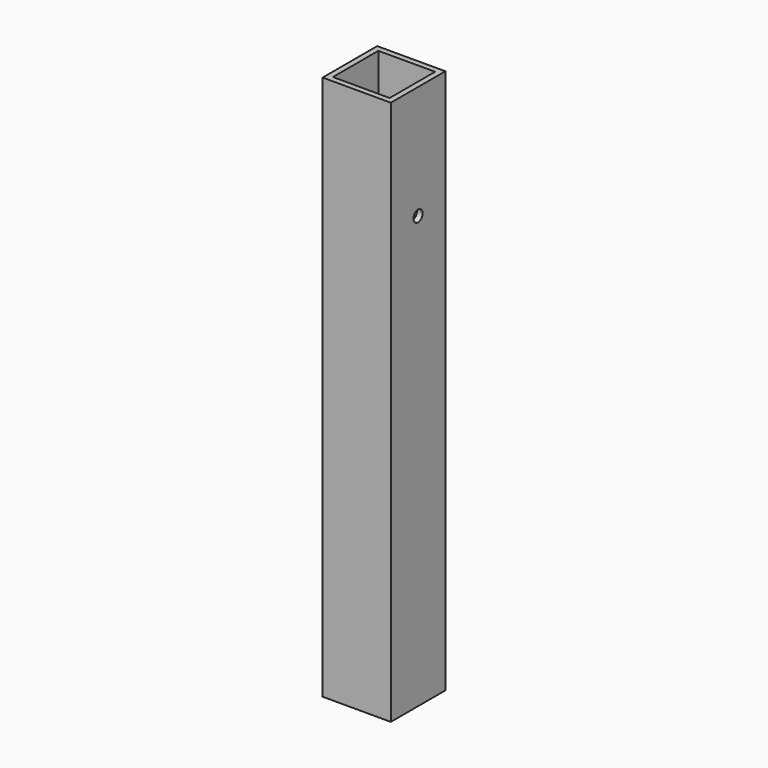
from build123d import *

# Parameters (mm, degrees)
F0_W     = 76.2
F0_H     = 76.2
F0_W_2   = 63.5
F0_H_2   = 63.5
F1_DEPTH = 609.6
F3_D     = 12.7


# Not quite as in the source:
# - a length typed as a fraction of an inch, garbled in the dataset ("3 / 203.2 mm" for 3/8 in), is restored


with BuildPart() as f1:
    # F0 (on Top) → F1 (new body)
    with BuildSketch(Plane.XY):
        Rectangle(F0_W, F0_H)
        Rectangle(F0_W_2, F0_H_2, mode=Mode.SUBTRACT)
    extrude(amount=F1_DEPTH)

    # F3 (through all)
    with Locations(Plane.YZ.offset(38.1)):
        with Locations((0, 482.6)):
            Hole(F3_D / 2)


solid = f1.part
